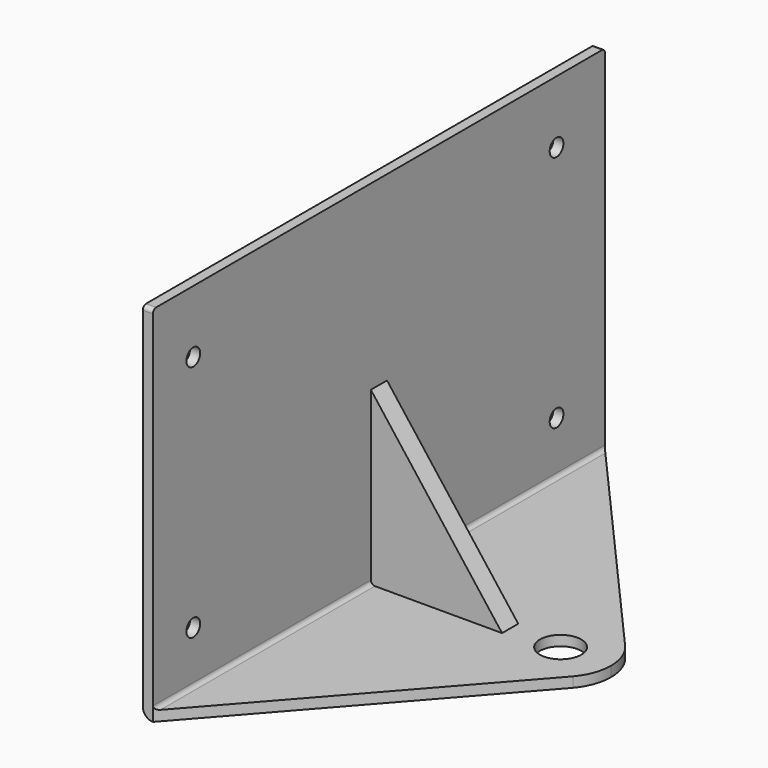
from build123d import *

# Parameters (mm, degrees)
F1_DEPTH  = 280
F2_R      = 2
F3_R      = 4.25
F4_DEPTH  = 5.001
F5_W      = 10
F5_H      = 85
F6_DEPTH  = 65
F8_DEPTH  = 145.001
F9_R      = 10.25
F10_DEPTH = 5.001
F11_R     = 5
F12_R     = 2


# Not quite as in the source:
# - a feature names something its author has since deleted; it is built from what else it names


with BuildPart() as f1:
    # F0 (on Front) → F1 (new body)
    with BuildSketch(Plane.XZ):
        Polygon((0, 87.5), (-5, 87.5), (-5, -92.5), (115, -92.5), (115, -87.5), (0, -87.5), align=None)
    extrude(amount=-F1_DEPTH)

    # F2
    f2_edges = [f1.edges().sort_by_distance(p)[0] for p in [
        (-2.5, 280, 87.5),
        (-2.5, 0, 87.5),
    ]]
    fillet(f2_edges, radius=F2_R)

    # F3 (on face) → F4 (cut, through all)
    with BuildSketch(Plane.YZ):
        with Locations((25, 56.5)):
            Circle(F3_R)
        with Locations((25, -61.5)):
            Circle(F3_R)
        with Locations((250, -61.5)):
            Circle(F3_R)
        with Locations((250, 56.5)):
            Circle(F3_R)
    extrude(amount=-F4_DEPTH, mode=Mode.SUBTRACT)

    # F5 (on face) → F6 (join)
    with BuildSketch(Plane.YZ):
        with Locations((140, -45)):
            Rectangle(F5_W, F5_H)
    extrude(amount=F6_DEPTH)

    # F7 (on face) → F8 (cut, through all)
    with BuildSketch(Plane(origin=(0, 145, 0), x_dir=(-1, 0, 0), z_dir=(0, 1, 0))):
        Polygon((-65, -87.5), (0, -2.5), (-65, -2.5), align=None)
    extrude(amount=-F8_DEPTH, mode=Mode.SUBTRACT)

    # F9 (on face) → F10 (cut, through all)
    with BuildSketch(Plane.XY.offset(-87.5)):
        with Locations((90, 140)):
            Circle(F9_R)
        with BuildLine():
            ThreePointArc((109.1388440622, 156.0842981806), (113.4890517215, 148.5594654753), (115, 140))
            Line((115, 140), (115, 280))
            Line((115, 280), (0, 280))
            Line((0, 280), (109.1388440622, 156.0842981806))
        make_face()
        with BuildLine():
            ThreePointArc((115, 140), (113.4890517215, 131.4405345247), (109.1388440622, 123.9157018194))
            Line((109.1388440622, 123.9157018194), (0, 0))
            Line((0, 0), (115, 0))
            Line((115, 0), (115, 140))
        make_face()
    extrude(amount=-F10_DEPTH, mode=Mode.SUBTRACT)

    # F11
    f11_edges = [f1.edges().sort_by_distance(p)[0] for p in [
        (-5, 140, -92.5),
    ]]
    fillet(f11_edges, radius=F11_R)

    # F12
    f12_edges = [f1.edges().sort_by_distance(p)[0] for p in [
        (0, 212.5, -87.5),
        (0, 67.5, -87.5),
    ]]
    fillet(f12_edges, radius=F12_R)


solid = f1.part
